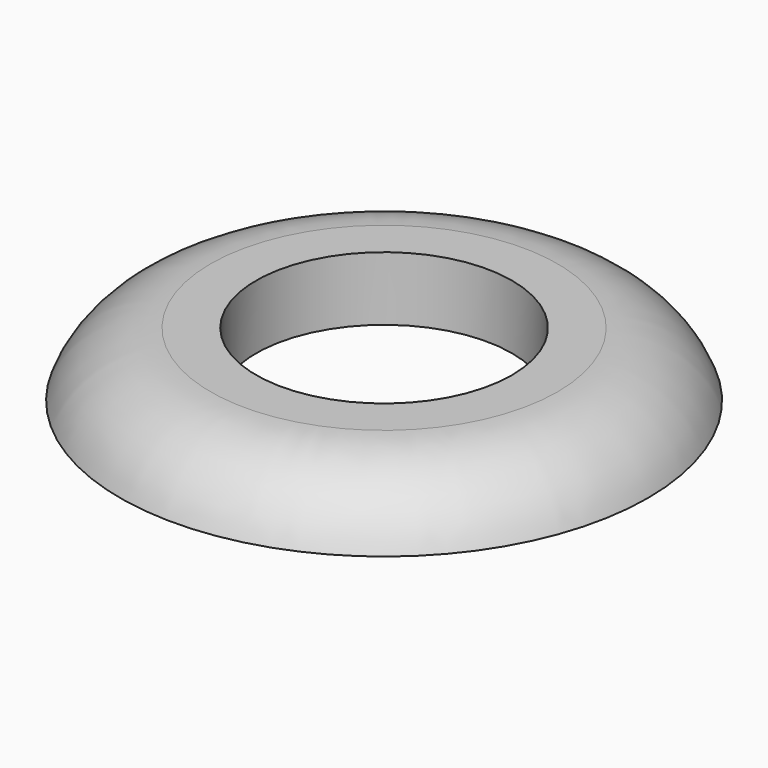
from build123d import *

# Parameters (mm, degrees)
F0_R     = 8.25
F0_R_2   = 4
F1_DEPTH = 2
F2_DEPTH = 2


# Not quite as in the source:
# - a fillet or chamfer that OpenCascade refuses, or shapes differently, is made with other operations: its cross-section is extruded or revolved along the edge and cut away or added


with BuildPart() as f1:
    # F0 (on Top) → F1 (new body)
    with BuildSketch(Plane.XY):
        Circle(F0_R)
        Circle(F0_R_2, mode=Mode.SUBTRACT)
        Circle(F0_R_2)
    extrude(amount=F1_DEPTH)

    # F0 (on Top) → F2 (cut, through all)
    with BuildSketch(Plane.XY):
        Circle(F0_R_2)
    extrude(amount=F2_DEPTH, mode=Mode.SUBTRACT)

    # F3: fillet of radius 3 on 1 edges, made by hand

    # F3_s1 → F3_t2 (revolve, cut)
    with BuildSketch(Plane.XZ):
        with BuildLine():
            ThreePointArc((8.25, 0), (7.1536236828, 1.4494897428), (5.4215728753, 2))
            Line((5.4215728753, 2), (8.25, 2))
            Line((8.25, 2), (8.25, 0))
        make_face()
    revolve(axis=Axis((0, 0, 2), (0, 0, 1)), mode=Mode.SUBTRACT)


solid = f1.part
